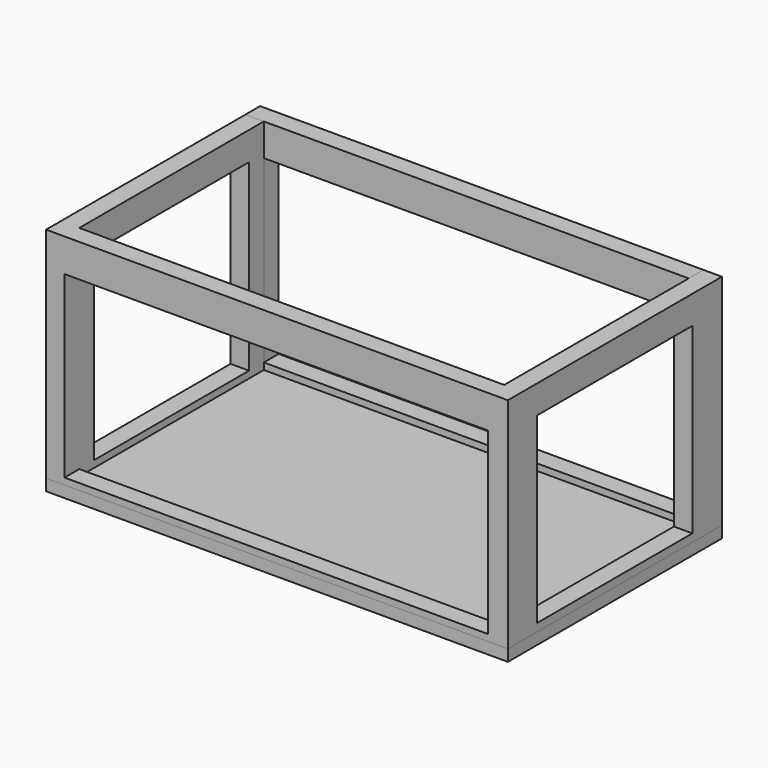
from build123d import *

# Parameters (mm, degrees)
F1_DEPTH  = 40
F2_DEPTH  = 40
F4_DEPTH  = 40
F5_W      = 1001.1475086212
F5_H      = 499.4027398658
F5_W_2    = 918.1282734871
F5_H_2    = 388.4018957615
F6_DEPTH  = 40
F7_W      = 580
F7_H      = 499.4027398658
F7_W_2    = 420.3874319792
F7_H_2    = 396.1715698242
F8_DEPTH  = 40
F9_W      = 1001.1475086212
F9_H      = 580
F10_DEPTH = 25


# Not quite as in the source:
# - a feature names something its author has since deleted; it is built from what else it names


with BuildPart() as f1:
    # F0 (on Front) → F1 (new body)
    with BuildSketch(Plane.XZ):
        Polygon((-500, 208.3333301377), (-500, 138.3333301377), (-460, 138.3333301377), (460, 138.3333301377), (500, 138.3333301377), (500, 208.3333301377), align=None)
        Polygon((-500, 138.3333301377), (-500, -291.6666698623), (500, -291.6666698623), (500, 138.3333301377), (460, 138.3333301377), (460, -251.6666698623), (-460, -251.6666698623), (-460, 138.3333301377), align=None)
    extrude(amount=F1_DEPTH)


with BuildPart() as f2:
    # F0 (on Front) → F2 (new body)
    with BuildSketch(Plane.XZ):
        Polygon((-500, 138.3333301377), (-500, -291.6666698623), (500, -291.6666698623), (500, 138.3333301377), (460, 138.3333301377), (460, -251.6666698623), (-460, -251.6666698623), (-460, 138.3333301377), align=None)
        Polygon((-500, 208.3333301377), (-500, 138.3333301377), (-460, 138.3333301377), (460, 138.3333301377), (500, 138.3333301377), (500, 208.3333301377), align=None)
    extrude(amount=F2_DEPTH)


with BuildPart() as f4:
    # F3 (on face) → F4 (new body)
    with BuildSketch(Plane(origin=(-500, 0, 0), x_dir=(0, -1, 0), z_dir=(-1, 0, 0))):
        Polygon((40, 208.3333301377), (40, 146.9305902719), (80, 146.9305902719), (500, 146.9305902719), (540, 146.9305902719), (540, 208.3333301377), align=None)
        Polygon((80, 146.9305902719), (40, 146.9305902719), (40, -291.0694097281), (540, -291.0694097281), (540, 146.9305902719), (500, 146.9305902719), (500, -251.0694097281), (80, -251.0694097281), align=None)
    extrude(amount=-F4_DEPTH)

    # F5 (on face) → F6 (join)
    with BuildSketch(Plane.XZ.offset(540)):
        with Locations((0.5737543106, -41.3680397952)):
            Rectangle(F5_W, F5_H)
        with Locations((-0.9358632565, -57.6452165842)):
            Rectangle(F5_W_2, F5_H_2, mode=Mode.SUBTRACT)
    extrude(amount=F6_DEPTH)

    # F7 (on face) → F8 (join)
    with BuildSketch(Plane.YZ.offset(501.1475086212)):
        with Locations((-290, -41.3680397952)):
            Rectangle(F7_W, F7_H)
        with Locations((-290.2767434716, -50.868704915)):
            Rectangle(F7_W_2, F7_H_2, mode=Mode.SUBTRACT)
    extrude(amount=-F8_DEPTH)


with BuildPart() as f10:
    # F9 (on face) → F10 (new body)
    with BuildSketch(Plane(origin=(0, 0, -291.0694097281), x_dir=(1, 0, 0), z_dir=(0, 0, -1))):
        with Locations((0.5737543106, 290)):
            Rectangle(F9_W, F9_H)
    extrude(amount=-F10_DEPTH)


solid = Compound([f1.part, f2.part, f4.part, f10.part])
